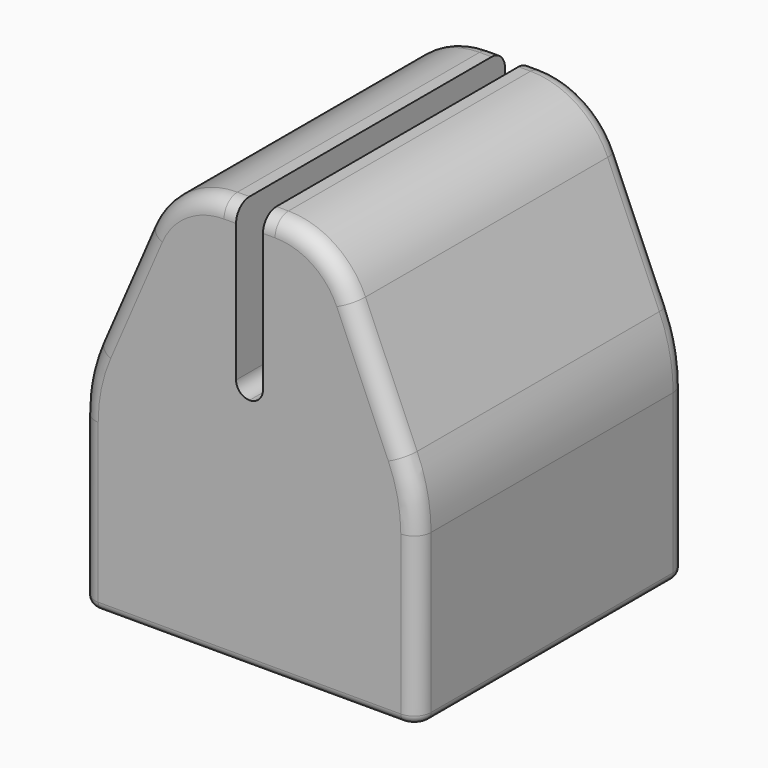
from build123d import *

# Parameters (mm, degrees)
F0_W     = 10
F0_H     = 12
F1_DEPTH = 10
F2_R     = 10
F3_R     = 5
F4_R     = 1
F5_R     = 0.79999
F6_R     = 0.5


# Not quite as in the source:
# - a fillet or chamfer is up to 0.001 mm smaller than in the source, because OpenCascade refuses the exact size
# - a feature names something its author has since deleted; it is built from what else it names


with BuildPart() as f1:
    # F0 (on Front) → F1 (new body, symmetric)
    with BuildSketch(Plane.XZ):
        Polygon((-0.8, 10), (-4.8, 10), (-10, -2), (0, -2), (0, 0), (-0.8, 0), align=None)
        Polygon((0, 0), (0, -2), (10, -2), (4.8, 10), (0.8, 10), (0.8, 0), align=None)
        with Locations((-5, -8)):
            Rectangle(F0_W, F0_H)
        with Locations((5, -8)):
            Rectangle(F0_W, F0_H)
    extrude(amount=F1_DEPTH, both=True)

    # F2
    f2_edges = [f1.edges().sort_by_distance(p)[0] for p in [
        (10, 0, -2),
        (-10, 0, -2),
    ]]
    fillet(f2_edges, radius=F2_R)

    # F3
    f3_edges = [f1.edges().sort_by_distance(p)[0] for p in [
        (4.8, 0, 10),
        (-4.8, 0, 10),
    ]]
    fillet(f3_edges, radius=F3_R)

    # F4
    f4_edges = [f1.edges().sort_by_distance(p)[0] for p in [
        (7.64037, 10, 3.4453),
        (7.64037, -10, 3.4453),
        (-7.64037, 10, 3.4453),
        (-7.64037, -10, 3.4453),
    ]]
    fillet(f4_edges, radius=F4_R)

    # F5 (radius 0.8 in the source; OpenCascade refuses exactly that, so slightly less here)
    f5_edges = [f1.edges().sort_by_distance(p)[0] for p in [
        (-0.8, 0, 0),
        (0.8, 0, 0),
    ]]
    fillet(f5_edges, radius=F5_R)

    # F6
    f6_edges = [f1.edges().sort_by_distance(p)[0] for p in [
        (-10, 0, -14),
        (-9.707107, 9.707107, -14),
        (-9.707107, -9.707107, -14),
        (0, 10, -14),
        (0, -10, -14),
        (9.707107, 9.707107, -14),
        (9.707107, -9.707107, -14),
        (10, 0, -14),
    ]]
    fillet(f6_edges, radius=F6_R)


solid = f1.part
